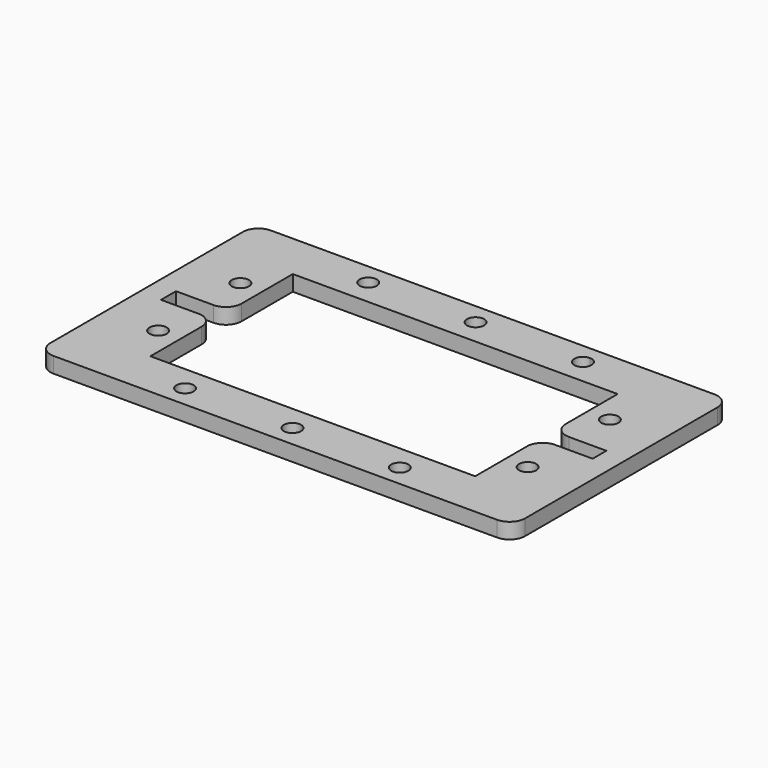
from build123d import *

# Parameters (mm, degrees)
F0_R     = 2.75
F1_DEPTH = 5


with BuildPart() as f1:
    # F0 (on Top) → F1 (new body)
    with BuildSketch(Plane.XY):
        with BuildLine():
            Line((0, 25.5), (0, 0))
            Line((0, 0), (14, 0))
            Line((14, 0), (14, 20.5))
            ThreePointArc((14, 20.5), (12.5355339059, 24.0355339059), (9, 25.5))
            Line((9, 25.5), (0, 25.5))
        make_face()
        with Locations((6.85, 12.05)):
            Circle(F0_R, mode=Mode.SUBTRACT)
        with BuildLine():
            Line((14, 0), (0, 0))
            Line((0, 0), (-10, 0))
            Line((-10, 0), (-10, -10))
            ThreePointArc((-10, -10), (-8.5355339059, -13.5355339059), (-5, -15))
            Line((-5, -15), (0, -15))
            Line((0, -15), (132, -15))
            Line((132, -15), (132, 0))
            Line((132, 0), (118, 0))
            Line((118, 0), (14, 0))
        make_face()
        with Locations((31.625, -8.15)):
            Circle(F0_R, mode=Mode.SUBTRACT)
        with Locations((66, -8.15)):
            Circle(F0_R, mode=Mode.SUBTRACT)
        with Locations((100.375, -8.15)):
            Circle(F0_R, mode=Mode.SUBTRACT)
        Polygon((-10, 0), (0, 0), (0, 25.5), (-3, 25.5), (-3, 28.5), (-3, 31.5), (0, 31.5), (0, 57), (-10, 57), align=None)
        with BuildLine():
            Line((118, 20.75), (118, 0))
            Line((118, 0), (132, 0))
            Line((132, 0), (132, 25.75))
            Line((132, 25.75), (123, 25.75))
            ThreePointArc((123, 25.75), (119.4644660941, 24.2855339059), (118, 20.75))
        make_face()
        with Locations((125.15, 12.05)):
            Circle(F0_R, mode=Mode.SUBTRACT)
        with BuildLine():
            Line((-10, 67), (-10, 57))
            Line((-10, 57), (0, 57))
            Line((0, 57), (0, 72))
            Line((0, 72), (-5, 72))
            ThreePointArc((-5, 72), (-8.5355339059, 70.5355339059), (-10, 67))
        make_face()
        with BuildLine():
            Line((0, 57), (0, 31.5))
            Line((0, 31.5), (9, 31.5))
            ThreePointArc((9, 31.5), (12.5355339059, 32.9644660941), (14, 36.5))
            Line((14, 36.5), (14, 57))
            Line((14, 57), (0, 57))
        make_face()
        with Locations((6.85, 44.95)):
            Circle(F0_R, mode=Mode.SUBTRACT)
        with BuildLine():
            Line((142, 0), (132, 0))
            Line((132, 0), (132, -15))
            Line((132, -15), (137, -15))
            ThreePointArc((137, -15), (140.5355339059, -13.5355339059), (142, -10))
            Line((142, -10), (142, 0))
        make_face()
        Polygon((132, 25.75), (132, 0), (142, 0), (142, 57), (132, 57), (132, 31.25), (135, 31.25), (135, 28.25), (135, 25.75), align=None)
        Polygon((0, 72), (0, 57), (14, 57), (118, 57), (132, 57), (132, 72), (100.375, 72), align=None)
        with Locations((31.625, 65.15)):
            Circle(F0_R, mode=Mode.SUBTRACT)
        with Locations((66, 65.15)):
            Circle(F0_R, mode=Mode.SUBTRACT)
        with BuildLine():
            ThreePointArc((103.125, 65.15), (98.4304563517, 63.2054563517), (100.375, 67.9))
            ThreePointArc((100.375, 67.9), (102.3195436483, 67.0945436483), (103.125, 65.15))
        make_face(mode=Mode.SUBTRACT)
        with BuildLine():
            Line((123, 31.25), (132, 31.25))
            Line((132, 31.25), (132, 57))
            Line((132, 57), (118, 57))
            Line((118, 57), (118, 36.25))
            ThreePointArc((118, 36.25), (119.4644660941, 32.7144660941), (123, 31.25))
        make_face()
        with Locations((125.15, 44.95)):
            Circle(F0_R, mode=Mode.SUBTRACT)
        with BuildLine():
            Line((132, 57), (142, 57))
            Line((142, 57), (142, 67))
            ThreePointArc((142, 67), (140.5355339059, 70.5355339059), (137, 72))
            Line((137, 72), (132, 72))
            Line((132, 72), (132, 57))
        make_face()
    extrude(amount=F1_DEPTH)


solid = f1.part
